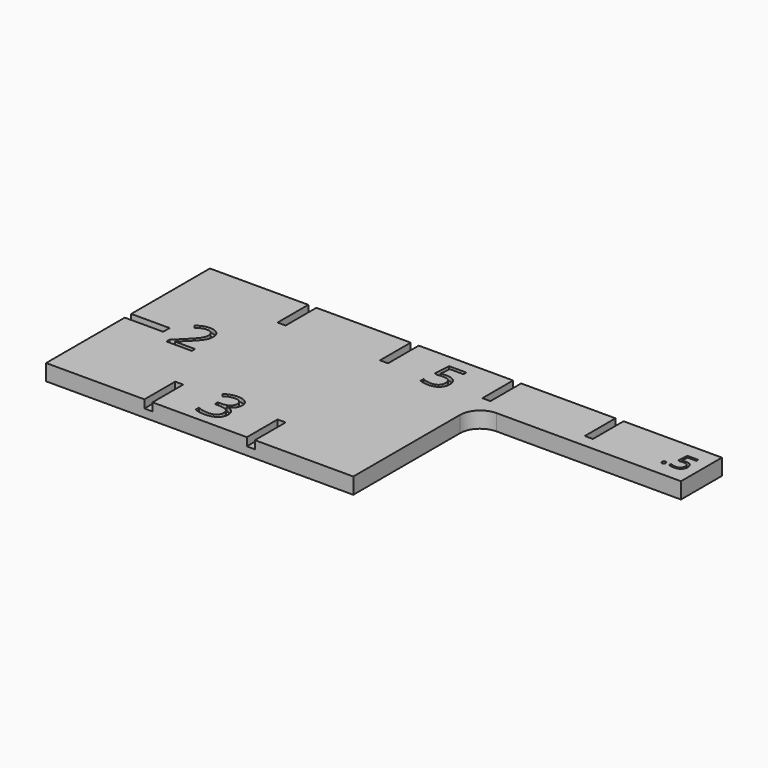
from build123d import *

# Parameters (mm, degrees)
F1_DEPTH       = 4
F2_W           = 2
F2_H           = 19.05
F2_W_2         = 19.05
F2_H_2         = 2
F3_DEPTH       = 2
F4_TEXT_SIZE   = 11.968633367
F4_TEXT_SIZE_2 = 13.4282240955
F4_TEXT_SIZE_3 = 13.4282250656
F4_TEXT_SIZE_4 = 7.589865062
F5_DEPTH       = 1


# Not quite as in the source:
# - Text() gives the source's letters only with a copy of the font that has no kerning and outlines rounded to 1/6400 em; it was checked with that copy


with BuildPart() as f1:
    # F0 (on Top) → F1 (new body)
    with BuildSketch(Plane.XY):
        with BuildLine():
            Line((-38.1, 25.4), (-38.1, -25.4))
            Line((-38.1, -25.4), (38.1, -25.4))
            Line((38.1, -25.4), (38.1, 7.7))
            ThreePointArc((38.1, 7.7), (39.5644660941, 11.2355339059), (43.1, 12.7))
            Line((43.1, 12.7), (88.9, 12.7))
            Line((88.9, 12.7), (88.9, 25.4))
            Line((88.9, 25.4), (-38.1, 25.4))
        make_face()
    extrude(amount=F1_DEPTH)

    # F2 (on face) → F3 (cut)
    with BuildSketch(Plane.XY.offset(4)):
        with Locations((-12.700015372, 25.4000279397)):
            Rectangle(F2_W, F2_H)
        with Locations((12.699984628, 25.4000279397)):
            Rectangle(F2_W, F2_H)
        with Locations((38.1, 25.4000279397)):
            Rectangle(F2_W, F2_H)
        with Locations((63.5, 25.4000276327)):
            Rectangle(F2_W, F2_H)
        with Locations((-38.1, 3.07e-07)):
            Rectangle(F2_W_2, F2_H_2)
        with Locations((-12.6998775363, -25.4)):
            Rectangle(F2_W, F2_H)
        with Locations((12.7001224637, -25.4)):
            Rectangle(F2_W, F2_H)
    extrude(amount=-F3_DEPTH, mode=Mode.SUBTRACT)

    # F4 (on face) → F5 (cut)
    with BuildSketch(Plane.XY.offset(4)):
        with Locations((22.4128253758, 13.7892942876)):
            Text('5', F4_TEXT_SIZE, font='Open Sans', text_align=(TextAlign.LEFT, TextAlign.BOTTOM))
        with Locations((-3.9130728692, -22.9189004749)):
            Text('3', F4_TEXT_SIZE_2, font='Open Sans', text_align=(TextAlign.LEFT, TextAlign.BOTTOM))
        with Locations((-26.1922497302, -3.7924384233)):
            Text('2', F4_TEXT_SIZE_3, font='Open Sans', text_align=(TextAlign.LEFT, TextAlign.BOTTOM))
        with Locations((80.3694725037, 16.3849294186)):
            Text('.5', F4_TEXT_SIZE_4, font='Open Sans', text_align=(TextAlign.LEFT, TextAlign.BOTTOM))
    extrude(amount=-F5_DEPTH, mode=Mode.SUBTRACT)


solid = f1.part
